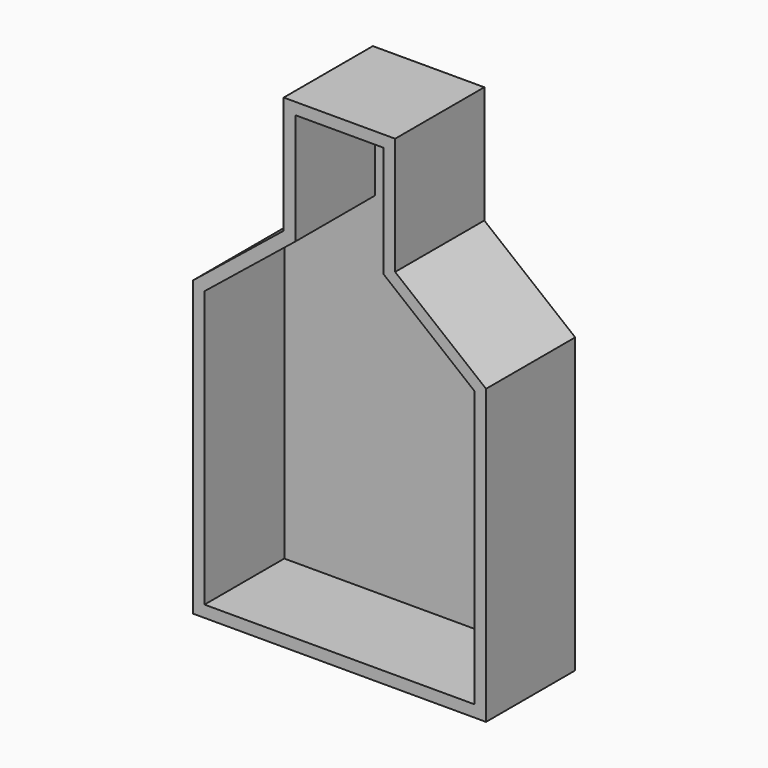
from build123d import *

# Parameters (mm, degrees)
F1_DEPTH = 19
F2_T     = -4


with BuildPart() as f1:
    # F0 (on Front) → F1 (new body, symmetric)
    with BuildSketch(Plane.XZ):
        Polygon((-50, 25), (-50, -75), (50, -75), (50, 25), (19, 50), (19, 90), (-19, 90), (-19, 50), align=None)
    extrude(amount=F1_DEPTH, both=True)

    # F2
    f2_openings = [f1.faces().sort_by_distance(p)[0] for p in [
        (0, -19, -6.201711),
    ]]
    offset(amount=F2_T, openings=f2_openings, kind=Kind.INTERSECTION)


solid = f1.part
